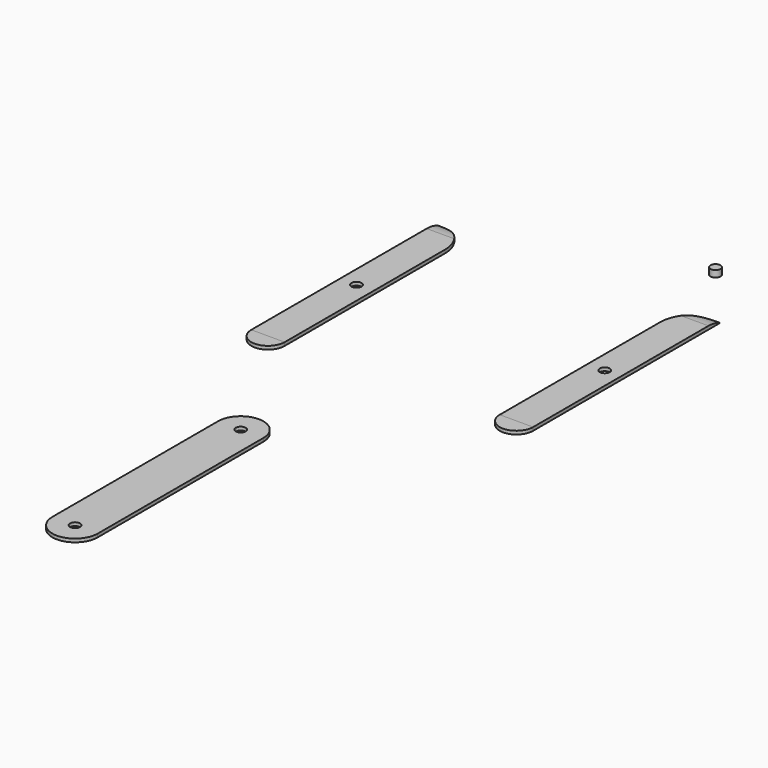
from build123d import *

# Parameters (mm, degrees)
F0_W        = 10
F0_H        = 70
F1_DEPTH    = 1
F2_T1_DEPTH = 51
F2_T3_DEPTH = 31.7944947177
F3_W        = 10
F3_H        = 70
F4_DEPTH    = 1
F5_T1_DEPTH = 51
F5_T3_DEPTH = 31.7944947177
F7_D        = 3
F10_D       = 3
F11_R       = 1.5
F12_DEPTH   = 2
F13_R       = 1.5
F14_DEPTH   = 1
F15_DEPTH   = 1
F16_DEPTH   = 1


# Not quite as in the source:
# - a fillet or chamfer that OpenCascade refuses, or shapes differently, is made with other operations: its cross-section is extruded or revolved along the edge and cut away or added


with BuildPart() as f1:
    # F0 (on Top) → F1 (new body)
    with BuildSketch(Plane.XY):
        with Locations((-38.6043904229, -0.6076917052)):
            Rectangle(F0_W, F0_H)
    extrude(amount=F1_DEPTH)

    # F2: fillet of radius 10 on 2 edges, made by hand

    # F2_s2 → F2_t1 (cut)
    with BuildSketch(Plane.XY.offset(-25)):
        with BuildLine():
            ThreePointArc((-33.6043904229, 24.3923082948), (-36.5333226111, 31.4633761066), (-43.6043904229, 34.3923082948))
            Line((-43.6043904229, 34.3923082948), (-33.6043904229, 34.3923082948))
            Line((-33.6043904229, 34.3923082948), (-33.6043904229, 24.3923082948))
        make_face()
    extrude(amount=F2_T1_DEPTH, mode=Mode.SUBTRACT)

    # F2_s4 → F2_t3 (cut)
    with BuildSketch(Plane.YZ.offset(-54.5016377818)):
        with BuildLine():
            ThreePointArc((34.3923082948, 0), (32.2694773287, 0.7467943448), (30.0334093512, 1))
            Line((30.0334093512, 1), (34.3923082948, 1))
            Line((34.3923082948, 1), (34.3923082948, 0))
        make_face()
    extrude(amount=F2_T3_DEPTH, mode=Mode.SUBTRACT)

    # F10 (through all)
    with Locations(Plane.XY.offset(1)):
        with Locations((-38.6452153325, -2.4311314337)):
            Hole(F10_D / 2)


with BuildPart() as f4:
    # F3 (on Top) → F4 (new body)
    with BuildSketch(Plane.XY):
        with Locations((33.6192296806, 2.1030642092)):
            Rectangle(F3_W, F3_H)
    extrude(amount=F4_DEPTH)

    # F5: fillet of radius 10 on 2 edges, made by hand

    # F5_s2 → F5_t1 (cut)
    with BuildSketch(Plane.XY.offset(-25)):
        with BuildLine():
            ThreePointArc((38.6192296806, 37.1030642092), (31.5481618688, 34.1741320211), (28.6192296806, 27.1030642092))
            Line((28.6192296806, 27.1030642092), (28.6192296806, 37.1030642092))
            Line((28.6192296806, 37.1030642092), (38.6192296806, 37.1030642092))
        make_face()
    extrude(amount=F5_T1_DEPTH, mode=Mode.SUBTRACT)

    # F5_s4 → F5_t3 (cut)
    with BuildSketch(Plane.YZ.offset(17.7219823218)):
        with BuildLine():
            ThreePointArc((37.1030642092, 0), (34.9802332432, 0.7467943448), (32.7441652657, 1))
            Line((32.7441652657, 1), (37.1030642092, 1))
            Line((37.1030642092, 1), (37.1030642092, 0))
        make_face()
    extrude(amount=F5_T3_DEPTH, mode=Mode.SUBTRACT)

    # F7 (through all)
    with Locations(Plane.XY.offset(1)):
        with Locations((33.7435789406, 0)):
            Hole(F7_D / 2)


with BuildPart() as f12:
    # F11 (on Top) → F12 (new body)
    with BuildSketch(Plane.XY):
        with Locations((22.5139018148, 55.5035099387)):
            Circle(F11_R)
    extrude(amount=F12_DEPTH)


with BuildPart() as f14:
    # F13 (on Top) → F14 (new body)
    with BuildSketch(Plane.XY):
        with BuildLine():
            ThreePointArc((-7.182598114, -76.6095072031), (-13.9708667994, -69.8212385178), (-20.7591354847, -76.6095072031))
            Line((-20.7591354847, -76.6095072031), (-20.7591354847, -138.6089920998))
            ThreePointArc((-20.7591354847, -138.6089920998), (-13.9708667994, -145.3972607851), (-7.182598114, -138.6089920998))
            Line((-7.182598114, -138.6089920998), (-7.182598114, -76.6095072031))
        make_face()
        with Locations((-13.9708667994, -138.6089920998)):
            Circle(F13_R, mode=Mode.SUBTRACT)
        with Locations((-13.9708667994, -76.6095072031)):
            Circle(F13_R, mode=Mode.SUBTRACT)
    extrude(amount=F14_DEPTH)


with BuildPart() as f15:
    # F6 (on face) → F15 (new body)
    with BuildSketch(Plane.XY.offset(1)):
        with BuildLine():
            Line((38.6192296806, -32.8969357908), (28.6192296806, -32.8969357908))
            ThreePointArc((28.6192296806, -32.8969357908), (33.6192296806, -37.8969357908), (38.6192296806, -32.8969357908))
        make_face()
    extrude(amount=-F15_DEPTH)


with BuildPart() as f16:
    # F8 (on face) → F16 (new body)
    with BuildSketch(Plane.XY.offset(1)):
        with BuildLine():
            ThreePointArc((-43.6043904229, -35.6076917052), (-38.6043904229, -40.6076917052), (-33.6043904229, -35.6076917052))
            Line((-33.6043904229, -35.6076917052), (-43.6043904229, -35.6076917052))
        make_face()
    extrude(amount=-F16_DEPTH)


solid = Compound([f1.part, f4.part, f12.part, f14.part, f15.part, f16.part])
